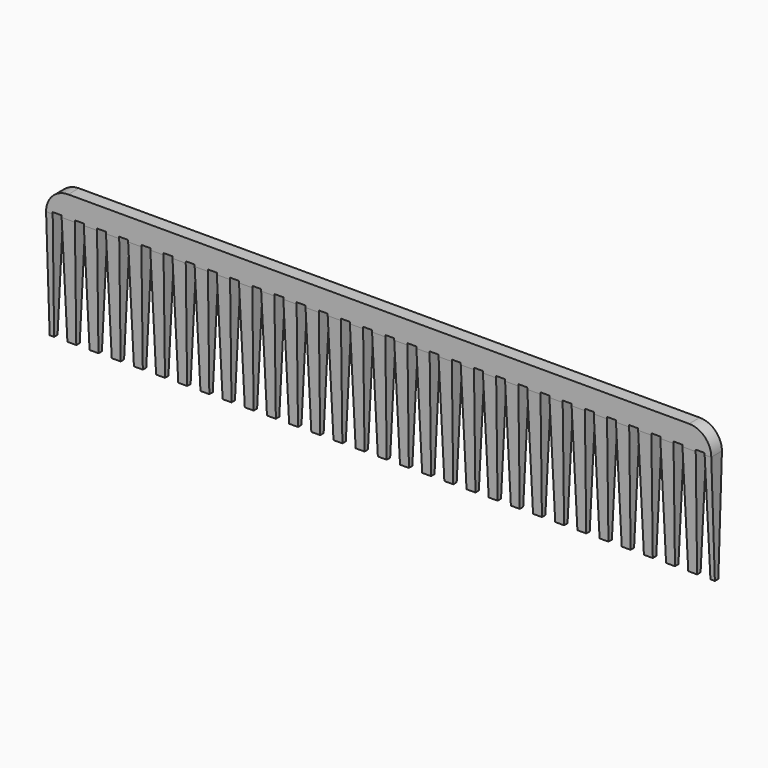
from build123d import *

# Parameters (mm, degrees)
F1_DEPTH = 1.5
F2_R     = 5
F5_DEPTH = 100


# Not quite as in the source:
# - a pattern or mirror of a feature is missing from the dataset's text; its kind, count and spacing are read off the source's solid


with BuildPart() as f1:
    # F0 (on Front) → F1 (new body, symmetric)
    with BuildSketch(Plane.XZ):
        Polygon((0, 30), (0, 0), (1, 0), (1.5, 25.3551919013), (3.5, 25.3551919013), (4, 0), (6, 0), (6.5, 25.3551919013), (8.5, 25.3551919013), (9, 0), (11, 0), (11.5, 25.3551919013), (13.5, 25.3551919013), (14, 0), (16, 0), (16.5, 25.3551919013), (18.5, 25.3551919013), (19, 0), (21, 0), (21.5, 25.3551919013), (23.5, 25.3551919013), (24, 0), (26, 0), (26.5, 25.3551919013), (28.5, 25.3551919013), (29, 0), (31, 0), (31.5, 25.3551919013), (33.5, 25.3551919013), (34, 0), (36, 0), (36.5, 25.3551919013), (38.5, 25.3551919013), (39, 0), (41, 0), (41.5, 25.3551919013), (43.5, 25.3551919013), (44, 0), (46, 0), (46.5, 25.3551919013), (48.5, 25.3551919013), (49, 0), (51, 0), (51.5, 25.3551919013), (53.5, 25.3551919013), (54, 0), (56, 0), (56.5, 25.3551919013), (58.5, 25.3551919013), (59, 0), (61, 0), (61.5, 25.3551919013), (63.5, 25.3551919013), (64, 0), (66, 0), (66.5, 25.3551919013), (68.5, 25.3551919013), (69, 0), (71, 0), (71.5, 25.3551919013), (73.5, 25.3551919013), (74, 0), (75, 0), (75, 30), align=None)
    extrude(amount=F1_DEPTH, both=True)

    # F2
    f2_edges = [f1.edges().sort_by_distance(p)[0] for p in [
        (75, 0, 30),
    ]]
    fillet(f2_edges, radius=F2_R)

    # F4: F1 across face


with BuildPart() as f1_1:
    add(f1.part)
    add(f1.part.mirror(Plane(origin=(0, 0, 15), x_dir=(0, -1, 0), z_dir=(-1, 0, 0))))

    # F3 (on Right) → F5 (cut, symmetric)
    with BuildSketch(Plane.YZ):
        Polygon((-0.48850436, 0), (-1.5, 24.95855093), (-1.5242770314, 0), align=None)
    f5 = extrude(amount=F5_DEPTH, both=True, mode=Mode.SUBTRACT)

    # F5_copies: F5 across plane
    add(f5.mirror(Plane.ZX), mode=Mode.SUBTRACT)


solid = f1_1.part
